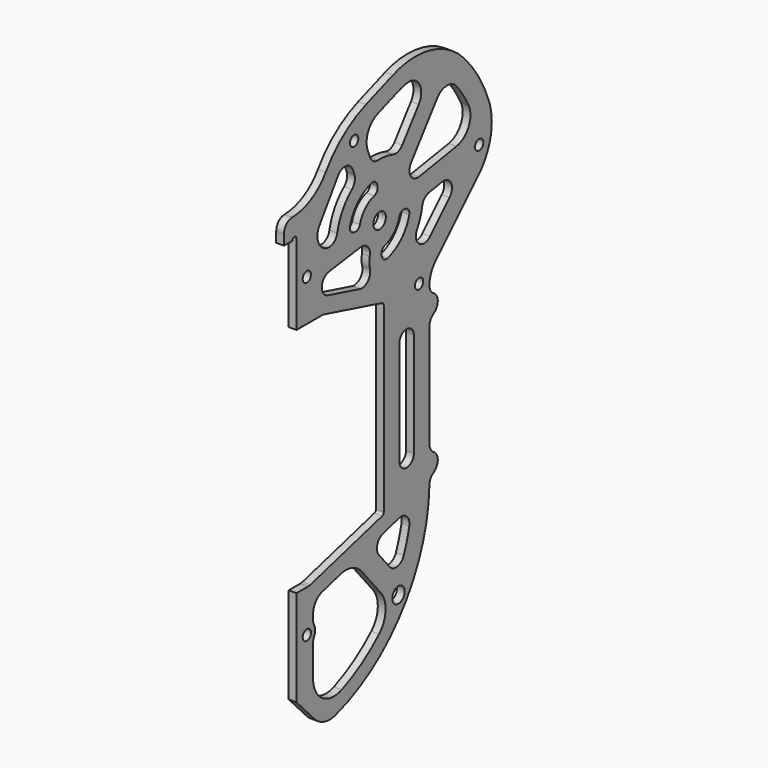
from build123d import *

# Parameters (mm, degrees)
F0_R     = 1
F0_R_2   = 1.5
F1_DEPTH = 1.5


# Not quite as in the source:
# - ends of sketch curves that miss each other by under 0.0002 mm in the source are joined


with BuildPart() as f1:
    # F0 (on Right) → F1 (new body)
    with BuildSketch(Plane.YZ):
        with BuildLine():
            Line((-21.996098, -27.31987), (-21.996098, -45.812627))
            Line((-21.996098, -45.812627), (-17.621845, -50.438265))
            ThreePointArc((-17.621845, -50.438265), (-15.2556042555, -51.8397305124), (-12.5061720552, -51.7778968223))
            ThreePointArc((-12.5061720552, -51.7778968223), (3.5454625901, -40.4951161641), (9.9951640259, -21.9652090006))
            ThreePointArc((9.9951640259, -21.9652090006), (10.2757378346, -20.9894720288), (10.9992601785, -20.2772223111))
            ThreePointArc((10.9992601785, -20.2772223111), (12.0039002073, -18.545177798), (11.0039019167, -16.8104491443))
            ThreePointArc((11.0039019167, -16.8104491443), (10.2718512165, -16.0783980417), (10.003902, -15.078398))
            Line((10.003902, -15.078398), (10.003902, 4.921602))
            ThreePointArc((10.003902, 4.921602), (10.2718512165, 5.9216020417), (11.0039020833, 6.6536528557))
            ThreePointArc((11.0039020833, 6.6536528557), (12.003902, 8.3856934558), (11.0039201798, 10.1177443114))
            ThreePointArc((11.0039201798, 10.1177443114), (10.269458941, 10.8540026976), (10.0039615857, 11.8594979972))
            ThreePointArc((10.0039615857, 11.8594979972), (10.3891645141, 13.7598432984), (11.4683680941, 15.3707479059))
            Line((11.4683680941, 15.3707479059), (21.774273, 25.676653))
            ThreePointArc((21.774273, 25.676653), (24.7317604297, 31.0578388491), (24.3439893135, 37.185932113))
            ThreePointArc((24.3439893135, 37.185932113), (21.7900626838, 42.4607965791), (18.1940737554, 47.088495765))
            ThreePointArc((18.1940737554, 47.088495765), (10.2755723108, 51.5882270472), (1.1845109874, 51.0379080347))
            Line((1.1845109874, 51.0379080347), (-5.280894, 48.684693))
            ThreePointArc((-5.280894, 48.684693), (-10.7177919764, 45.6790606822), (-14.9701240908, 41.1501140619))
            ThreePointArc((-14.9701240908, 41.1501140619), (-18.4726000988, 37.9865656192), (-23.0359049993, 36.7817319627))
            ThreePointArc((-23.0359049993, 36.7817319627), (-24.4243161193, 36.1821969282), (-24.996098, 34.782128))
            Line((-24.996098, 34.782128), (-24.996098, 32.779751))
            Line((-24.996098, 32.779751), (-22.996098, 32.779751))
            ThreePointArc((-22.996098, 32.779751), (-22.496098, 33.279751), (-21.996098, 32.779751))
            Line((-21.996098, 32.779751), (-21.996098, 17.279751))
            Line((-21.996098, 17.279751), (-15.831989, 17.279751))
            ThreePointArc((-15.831989, 17.279751), (-15.570936575, 17.2626407174), (-15.3143508308, 17.2116026314))
            Line((-15.3143508308, 17.2116026314), (-1.366688, 13.474338))
            ThreePointArc((-1.366688, 13.474338), (-1.0994211963, 13.2957555405), (-0.996098, 12.991375))
            Line((-0.996098, 12.991375), (-0.996098, -22.132359))
            ThreePointArc((-0.996098, -22.132359), (-1.0994211963, -22.4367395405), (-1.3666880537, -22.6153217996))
            Line((-1.3666880537, -22.6153217996), (-18.669968, -27.251722))
            ThreePointArc((-18.669968, -27.251722), (-18.9265537033, -27.3027597343), (-19.187606, -27.31987))
            Line((-19.187606, -27.31987), (-21.996098, -27.31987))
        make_face()
        with Locations((-19.496098, -35.419491)):
            Circle(F0_R, mode=Mode.SUBTRACT)
        with BuildLine():
            ThreePointArc((-17.7460980692, -36.3877369617), (-17.496098, -35.419491), (-17.7460980692, -34.4512450383))
            ThreePointArc((-17.7460980692, -34.4512450383), (-17.9325896552, -33.9829990692), (-17.996098, -33.482999))
            Line((-17.996098, -33.482999), (-17.996098, -32.478968))
            ThreePointArc((-17.996098, -32.478968), (-17.3761580188, -30.6526837103), (-15.7725551288, -29.5811905194))
            Line((-15.7725551288, -29.5811905194), (-11.424682, -28.416182))
            ThreePointArc((-11.424682, -28.416182), (-8.6270574238, -28.4772261134), (-6.3003638496, -30.0318728738))
            Line((-6.3003638496, -30.0318728738), (-1.723529, -35.486332))
            ThreePointArc((-1.723529, -35.486332), (-0.5624401991, -38.9949163794), (-2.1282627813, -42.3425262325))
            ThreePointArc((-2.1282627813, -42.3425262325), (-6.3573337492, -45.6393399924), (-11.1210981684, -48.1011625838))
            ThreePointArc((-11.1210981684, -48.1011625838), (-15.7911829634, -47.6118199936), (-17.996098, -43.466039))
            Line((-17.996098, -43.466039), (-17.996098, -37.355982))
            ThreePointArc((-17.996098, -37.355982), (-17.9325897646, -36.8559823544), (-17.7460980692, -36.3877369617))
        make_face(mode=Mode.SUBTRACT)
        with Locations((2.550308, -37.579716)):
            Circle(F0_R_2, mode=Mode.SUBTRACT)
        with BuildLine():
            Line((0.417191, -31.973043), (-2.175306, -28.883425))
            ThreePointArc((-2.175306, -28.883425), (-2.5506520894, -26.9964379968), (-1.1608561692, -25.6659973686))
            Line((-1.1608561692, -25.6659973686), (2.673734, -24.638522))
            ThreePointArc((2.673734, -24.638522), (4.5680584745, -25.1196037387), (5.1476802368, -26.9861360503))
            ThreePointArc((5.1476802368, -26.9861360503), (4.5711819336, -29.2325622712), (3.8091151123, -31.4230040444))
            ThreePointArc((3.8091151123, -31.4230040444), (2.2694207433, -32.6616792107), (0.417191, -31.973043))
        make_face(mode=Mode.SUBTRACT)
        with BuildLine():
            Line((2.753902, -15.078398), (2.753902, 4.921602))
            ThreePointArc((2.753902, 4.921602), (4.503902, 6.671602), (6.253902, 4.921602))
            Line((6.253902, 4.921602), (6.253902, -15.078398))
            ThreePointArc((6.253902, -15.078398), (4.503902, -16.828398), (2.753902, -15.078398))
        make_face(mode=Mode.SUBTRACT)
        with Locations((-19.496098, 25.279751)):
            Circle(F0_R, mode=Mode.SUBTRACT)
        with BuildLine():
            Line((-6.767723, 18.027369), (-14.425805, 20.079346))
            ThreePointArc((-14.425805, 20.079346), (-15.9042612839, 22.1361274193), (-14.1808899041, 23.992515303))
            Line((-14.1808899041, 23.992515303), (-6.577551, 25.039093))
            ThreePointArc((-6.577551, 25.039093), (-4.8203932786, 24.3980923464), (-4.3615548361, 22.5848209601))
            ThreePointArc((-4.3615548361, 22.5848209601), (-4.477484693, 21.5402984379), (-4.3247299968, 20.5005230009))
            ThreePointArc((-4.3247299968, 20.5005230009), (-4.8272219648, 18.553710138), (-6.767723, 18.027369))
        make_face(mode=Mode.SUBTRACT)
        with BuildLine():
            ThreePointArc((-14.5567540245, 28.1495958796), (-16.7346535441, 29.9536300539), (-16.4449966717, 32.7667927786))
            Line((-16.4449966717, 32.7667927786), (-12.351599, 38.835505))
            ThreePointArc((-12.351599, 38.835505), (-12.1477989547, 39.1318667137), (-11.9387027549, 39.4245158215))
            ThreePointArc((-11.9387027549, 39.4245158215), (-10.058959181, 40.2298668034), (-8.4541402996, 38.9623558853))
            Line((-8.4541402996, 38.9623558853), (-8.060642, 37.934613))
            ThreePointArc((-8.060642, 37.934613), (-7.9933516406, 36.7140017623), (-8.6490128126, 35.6822417749))
            ThreePointArc((-8.6490128126, 35.6822417749), (-10.9344787533, 33.0050906706), (-12.1959899918, 29.7188949984))
            ThreePointArc((-12.1959899918, 29.7188949984), (-13.050327583, 28.4437625647), (-14.5567540245, 28.1495958796))
        make_face(mode=Mode.SUBTRACT)
        with BuildLine():
            ThreePointArc((-8.3564720989, 28.2540276311), (-9.0243989567, 28.7665460217), (-9.1342894359, 29.6012468489))
            ThreePointArc((-9.1342894359, 29.6012468489), (-7.221617113, 32.914093113), (-3.9087709469, 34.8267658017))
            ThreePointArc((-3.9087709469, 34.8267658017), (-3.0740700217, 34.7168759567), (-2.5615515641, 34.0489488489))
            Line((-2.5615515641, 34.0489488489), (-2.486494, 33.76883))
            ThreePointArc((-2.486494, 33.76883), (-2.5963839786, 32.9341291338), (-3.2643109011, 32.4216106311))
            ThreePointArc((-3.2643109011, 32.4216106311), (-5.4609207948, 31.1533976608), (-6.7291343423, 28.9567880917))
            ThreePointArc((-6.7291343423, 28.9567880917), (-7.2416529097, 28.288861108), (-8.0763538489, 28.1789705641))
            Line((-8.0763538489, 28.1789705641), (-8.3564720989, 28.2540276311))
        make_face(mode=Mode.SUBTRACT)
        with Locations((-1.996098, 27.688574)):
            Circle(F0_R_2, mode=Mode.SUBTRACT)
        with Locations((-8.121383, 43.686669)):
            Circle(F0_R, mode=Mode.SUBTRACT)
        with BuildLine():
            Line((-1.430644, 21.3282), (-1.505702, 21.608318))
            ThreePointArc((-1.505702, 21.608318), (-1.3958117152, 22.4430193965), (-0.7278839158, 22.9555376859))
            ThreePointArc((-0.7278839158, 22.9555376859), (1.4687256608, 24.2237512052), (2.7369386593, 26.4203610913))
            ThreePointArc((2.7369386593, 26.4203610913), (3.2494571338, 27.0882880214), (4.0841580989, 27.1981783689))
            Line((4.0841580989, 27.1981783689), (4.364277, 27.123121))
            ThreePointArc((4.364277, 27.123121), (5.0322040214, 26.6106028662), (5.1420943689, 25.7759019011))
            ThreePointArc((5.1420943689, 25.7759019011), (3.229421546, 22.46305532), (-0.0834248031, 20.5503822653))
            ThreePointArc((-0.0834248031, 20.5503822653), (-0.9181258662, 20.6602729786), (-1.430644, 21.3282))
        make_face(mode=Mode.SUBTRACT)
        with Locations((7.503902, 13.146944)):
            Circle(F0_R, mode=Mode.SUBTRACT)
        with BuildLine():
            ThreePointArc((8.2610496287, 25.9707480622), (8.8217830592, 27.0570250546), (9.9099700271, 27.6140428345))
            Line((9.9099700271, 27.6140428345), (13.098357, 28.136825))
            ThreePointArc((13.098357, 28.136825), (15.2015024129, 27.0760034199), (14.8361780624, 24.7489659376))
            Line((14.8361780624, 24.7489659376), (10.150334, 20.063122))
            ThreePointArc((10.150334, 20.063122), (7.5177667465, 19.8912658497), (7.0051173965, 22.4791483493))
            ThreePointArc((7.0051173965, 22.4791483493), (7.7900633915, 24.1684823506), (8.2610496287, 25.9707480622))
        make_face(mode=Mode.SUBTRACT)
        with BuildLine():
            Line((-2.49442, 45.955934), (2.394616, 47.735397))
            ThreePointArc((2.394616, 47.735397), (3.4373252946, 48.0640337253), (4.5047620376, 48.3003037863))
            ThreePointArc((4.5047620376, 48.3003037863), (7.5818252173, 46.9139330558), (7.422211849, 43.5427511135))
            Line((7.422211849, 43.5427511135), (3.45896, 38.27169))
            ThreePointArc((3.45896, 38.27169), (2.4608377023, 37.5658778413), (1.2383930198, 37.5728080606))
            ThreePointArc((1.2383930198, 37.5728080606), (-0.5497351994, 37.9875076656), (-2.3829199888, 38.0813777001))
            ThreePointArc((-2.3829199888, 38.0813777001), (-3.5599861465, 38.4114308125), (-4.3250867004, 39.3648671147))
            Line((-4.3250867004, 39.3648671147), (-4.861895, 40.766909))
            ThreePointArc((-4.861895, 40.766909), (-4.7654691919, 43.8575037621), (-2.49442, 45.955934))
        make_face(mode=Mode.SUBTRACT)
        with BuildLine():
            ThreePointArc((11.859796151, 42.7887138865), (14.1961631415, 43.985186443), (16.5795798456, 42.8854218737))
            ThreePointArc((16.5795798456, 42.8854218737), (18.1256065821, 40.7697438525), (19.4317694803, 38.4981297378))
            ThreePointArc((19.4317694803, 38.4981297378), (19.4257656197, 34.8830903624), (16.5076749457, 32.7492453311))
            Line((16.5076749457, 32.7492453311), (7.512064, 31.274283))
            ThreePointArc((7.512064, 31.274283), (5.4774784003, 32.2122847196), (5.5899054074, 34.4498604456))
            Line((5.5899054074, 34.4498604456), (11.859796151, 42.7887138865))
        make_face(mode=Mode.SUBTRACT)
        with Locations((21.958067, 30.811764)):
            Circle(F0_R, mode=Mode.SUBTRACT)
    extrude(amount=F1_DEPTH)


solid = f1.part
